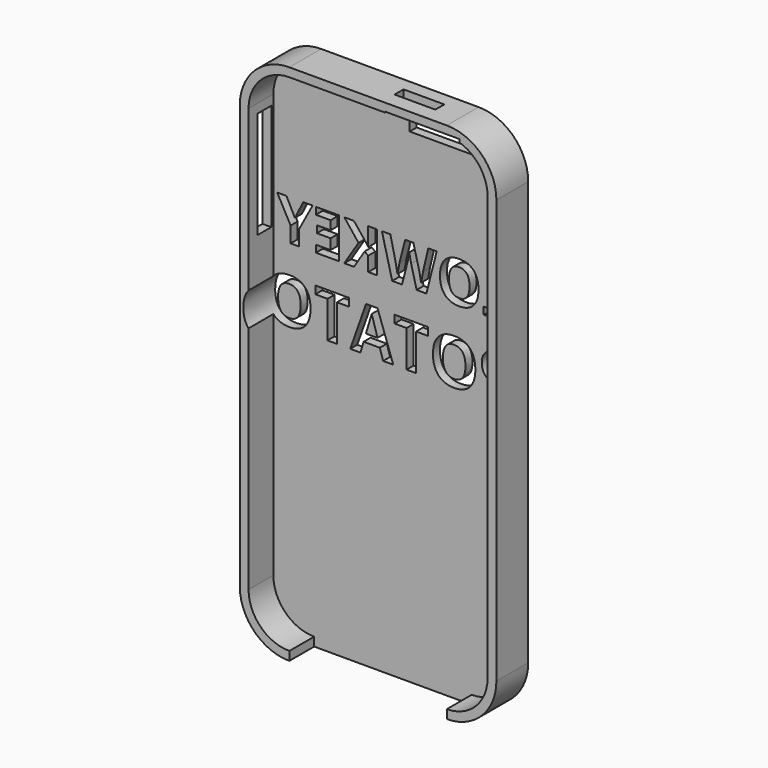
from build123d import *

# Parameters (mm, degrees)
F1_DEPTH       = 7.6
F2_T           = 2.15
F3_W           = 38.6
F3_H           = 7.6
F4_DEPTH       = 50.72
F5_W           = 18.3
F5_H           = 7.4
F6_DEPTH       = 18.3
F7_W           = 4.2
F7_H           = 26.2
F8_DEPTH       = 26.6
F10_W          = 0.6246941544
F10_H          = 2.7586207226
F10_W_2        = 9.3753058456
F11_DEPTH      = 10
F9_TEXT_SIZE   = 13.8888888889
F9_TEXT_SIZE_2 = 15.2777777778
F12_DEPTH      = 25


# Not quite as in the source:
# - Text() gives the source's letters only with a copy of the font that has no kerning and outlines rounded to 1/6400 em; it was checked with that copy


with BuildPart() as f1:
    # F0 (on Front) → F1 (new body)
    with BuildSketch(Plane.XZ):
        with BuildLine():
            Line((20.2810919291, 53.1843451649), (-38.3189080709, 53.1843451649))
            Line((-38.3189080709, 53.1843451649), (-38.3189080709, -50.6156548351))
            ThreePointArc((-38.3189080709, -50.6156548351), (-35.3899758828, -57.686722647), (-28.3189080709, -60.6156548351))
            Line((-28.3189080709, -60.6156548351), (10.2810919291, -60.6156548351))
            ThreePointArc((10.2810919291, -60.6156548351), (17.3521597409, -57.686722647), (20.2810919291, -50.6156548351))
            Line((20.2810919291, -50.6156548351), (20.2810919291, 53.1843451649))
        make_face()
        with BuildLine():
            Line((10.2810919291, 63.1843451649), (-28.3189080709, 63.1843451649))
            ThreePointArc((-28.3189080709, 63.1843451649), (-35.3899758828, 60.2554129768), (-38.3189080709, 53.1843451649))
            Line((-38.3189080709, 53.1843451649), (20.2810919291, 53.1843451649))
            ThreePointArc((20.2810919291, 53.1843451649), (17.3521597409, 60.2554129768), (10.2810919291, 63.1843451649))
        make_face()
    extrude(amount=F1_DEPTH)

    # F2
    f2_openings = [f1.faces().sort_by_distance(p)[0] for p in [
        (-9.018908, -7.6, 1.284345),
    ]]
    offset(amount=F2_T, openings=f2_openings, kind=Kind.INTERSECTION)

    # F3 (on face) → F4 (cut)
    with BuildSketch(Plane(origin=(0, 0, -62.7656548351), x_dir=(1, 0, 0), z_dir=(0, 0, -1))):
        with Locations((-9.0189080709, 3.8)):
            Rectangle(F3_W, F3_H)
    extrude(amount=-F4_DEPTH, mode=Mode.SUBTRACT)

    # F5 (on face) → F6 (cut)
    with BuildSketch(Plane(origin=(0, 2.15, 0), x_dir=(-1, 0, 0), z_dir=(0, 1, 0))):
        with Locations((-4.2384474635, 59.6978485107)):
            Rectangle(F5_W, F5_H)
    extrude(amount=-F6_DEPTH, mode=Mode.SUBTRACT)

    # F7 (on face) → F8 (cut)
    with BuildSketch(Plane(origin=(-40.4689080709, 0, 0), x_dir=(0, -1, 0), z_dir=(-1, 0, 0))):
        with Locations((2.7458126853, 37.8643451649)):
            Rectangle(F7_W, F7_H)
    extrude(amount=-F8_DEPTH, mode=Mode.SUBTRACT)

    # F10 (on face) → F11 (cut)
    with BuildSketch(Plane.XY.offset(65.3343451649)):
        with Locations((-5.2238996137, -2.4706896387)):
            Rectangle(F10_W, F10_H)
        with Locations((-0.2238996137, -2.4706896387)):
            Rectangle(F10_W_2, F10_H)
    extrude(amount=-F11_DEPTH, mode=Mode.SUBTRACT)

    # F9 (on face) → F12 (cut)
    with BuildSketch(Plane(origin=(0, 2.15, 0), x_dir=(-1, 0, 0), z_dir=(0, 1, 0))):
        with Locations((-20.6191700086, 22.3669291394)):
            Text('LOWKEY', F9_TEXT_SIZE, font='Open Sans', font_style=FontStyle.BOLD, text_align=(TextAlign.LEFT, TextAlign.BOTTOM))
        with Locations((-21.6716506796, 4.3669117008)):
            Text('POTATO', F9_TEXT_SIZE_2, font='Open Sans', font_style=FontStyle.BOLD, text_align=(TextAlign.LEFT, TextAlign.BOTTOM))
    extrude(amount=-F12_DEPTH, mode=Mode.SUBTRACT)


solid = f1.part
